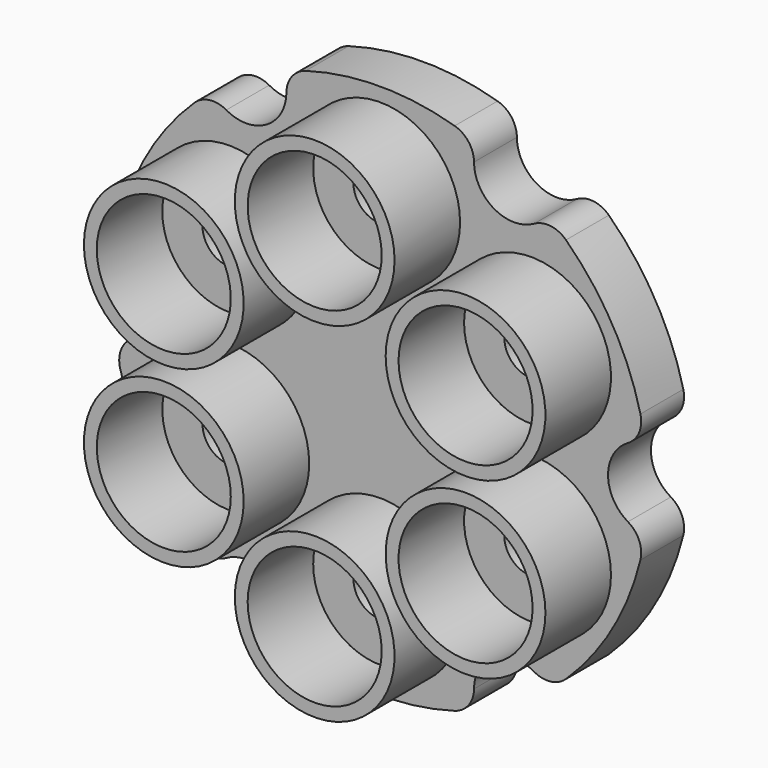
from build123d import *

# Parameters (mm, degrees)
F0_R            = 31.75
F1_DEPTH        = 6.35
F2_R            = 4.7625
F3_DEPTH        = 6.351
F3_COPIES_COUNT = 6
F4_R            = 3.175
F5_R            = 3.175
F6_DEPTH        = 6.3510001
F6_COPIES_COUNT = 6
F7_R            = 9.4615
F7_R_2          = 7.9375
F8_DEPTH        = 9.7028
F8_COPIES_COUNT = 6


# Not quite as in the source:
# - a pattern or mirror of a feature is missing from the dataset's text; its kind, count and spacing are read off the source's solid


with BuildPart() as f1:
    # F0 (on Front) → F1 (new body)
    with BuildSketch(Plane.XZ):
        Circle(F0_R)
    extrude(amount=F1_DEPTH)

    # F2 (on face) → F3 (cut, through all)
    with BuildSketch(Plane.XZ.offset(6.35)):
        with Locations((-15.875, 27.4963065702)):
            Circle(F2_R)
    f3 = extrude(amount=-F3_DEPTH, mode=Mode.SUBTRACT)

    # F3_copies: F3 ×6 about axis
    f3_copies_axis = Axis((0, 0, 0), (0, 1, 0))
    for i in range(1, F3_COPIES_COUNT):
        add(f3.rotate(f3_copies_axis, i * 360 / F3_COPIES_COUNT), mode=Mode.SUBTRACT)

    # F4
    f4_edges = [f1.edges().sort_by_distance(p)[0] for p in [
        (-19.809236, -3.175, 24.81243),
        (-11.583577, -3.175, 29.561516),
        (-31.392813, -3.175, 4.749087),
        (11.583577, -3.175, 29.561516),
        (19.809236, -3.175, 24.81243),
        (31.392813, -3.175, 4.749087),
        (31.392813, -3.175, -4.749087),
        (19.809236, -3.175, -24.81243),
        (11.583577, -3.175, -29.561516),
        (-11.583577, -3.175, -29.561516),
        (-19.809236, -3.175, -24.81243),
        (-31.392813, -3.175, -4.749087),
    ]]
    fillet(f4_edges, radius=F4_R)

    # F5 (on face) → F6 (cut, through all)
    with BuildSketch(Plane.XZ.offset(6.35)):
        with Locations((0, 20.6375)):
            Circle(F5_R)
    f6 = extrude(amount=-F6_DEPTH, mode=Mode.SUBTRACT)

    # F6_copies: F6 ×6 about axis
    f6_copies_axis = Axis((0, 0, 0), (0, 1, 0))
    for i in range(1, F6_COPIES_COUNT):
        add(f6.rotate(f6_copies_axis, i * 360 / F6_COPIES_COUNT), mode=Mode.SUBTRACT)

    # F7 (on face) → F8 (join)
    with BuildSketch(Plane.XZ.offset(6.35)):
        with Locations((0, 20.6375)):
            Circle(F7_R)
        with Locations((0, 20.6375)):
            Circle(F7_R_2, mode=Mode.SUBTRACT)
    f8 = extrude(amount=F8_DEPTH)

    # F8_copies: F8 ×6 about axis
    f8_copies_axis = Axis((0, 0, 0), (0, 1, 0))
    for i in range(1, F8_COPIES_COUNT):
        add(f8.rotate(f8_copies_axis, i * 360 / F8_COPIES_COUNT))


solid = f1.part
